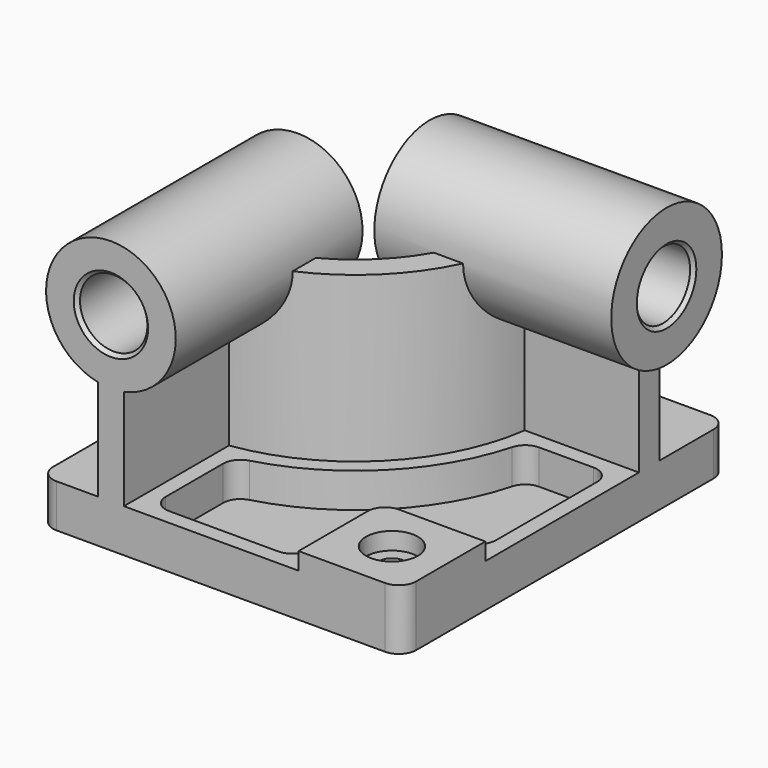
from build123d import *

# Parameters (mm, degrees)
F0_W            = 210
F0_H            = 225
F1_DEPTH        = 25
F3_DEPTH        = 95
F4_R            = 37.5
F5_DEPTH        = 10
F5_DEPTH_BACK   = 125
F6_R            = 40
F7_DEPTH        = 10
F7_DEPTH_BACK   = 127
F8_W            = 60
F8_H            = 60
F9_DEPTH        = 10
F10_R           = 10
F12_DEPTH       = 20
F14_D           = 15
F14_CBORE_D     = 30
F14_CBORE_DEPTH = 10
F15_R           = 10
F16_R           = 19.5
F17_DEPTH       = 235.001
F18_R           = 19.5
F19_DEPTH       = 220.001
F20_SIZE        = 2
F21_R           = 10


with BuildPart() as f1:
    # F0 (on Top) → F1 (new body)
    with BuildSketch(Plane.XY):
        Rectangle(F0_W, F0_H)
    extrude(amount=F1_DEPTH)

    # F2 (on face) → F3 (join)
    with BuildSketch(Plane.XY.offset(25)):
        with BuildLine():
            ThreePointArc((25, 63.5), (-3.1177490061, -4.3822509939), (-71, -32.5))
            Line((-71, -32.5), (-71, -112.5))
            Line((-71, -112.5), (-56, -112.5))
            Line((-56, -112.5), (-56, -46.4818166789))
            ThreePointArc((-56, -46.4818166789), (7.4888527117, -14.9888527117), (38.9818166789, 48.5))
            Line((38.9818166789, 48.5), (105, 48.5))
            Line((105, 48.5), (105, 63.5))
            Line((105, 63.5), (25, 63.5))
        make_face()
    extrude(amount=F3_DEPTH)

    # F4 (on face) → F5 (join, two sides)
    with BuildSketch(Plane.XZ.offset(112.5)) as f5_sk:
        with Locations((-63.5, 120)):
            Circle(F4_R)
        with BuildLine():
            ThreePointArc((-56, 83.2576538583), (-63.5, 82.5), (-71, 83.2576538583))
            Line((-71, 83.2576538583), (-71, 25))
            Line((-71, 25), (-105, 25))
            Line((-105, 25), (-105, 0))
            Line((-105, 0), (105, 0))
            Line((105, 0), (105, 25))
            Line((105, 25), (-56, 25))
            Line((-56, 25), (-56, 83.2576538583))
        make_face()
    extrude(amount=F5_DEPTH)
    extrude(f5_sk.sketch, amount=-F5_DEPTH_BACK)

    # F6 (on face) → F7 (join, two sides)
    with BuildSketch(Plane.YZ.offset(105)) as f7_sk:
        with Locations((56, 120)):
            Circle(F6_R)
        with BuildLine():
            ThreePointArc((63.5, 80.7094158862), (86.8220700148, 94.504902432), (96, 120))
            ThreePointArc((96, 120), (30.504902432, 150.8220700148), (48.5, 80.7094158862))
            Line((48.5, 80.7094158862), (48.5, 120))
            Line((48.5, 120), (63.5, 120))
            Line((63.5, 120), (63.5, 80.7094158862))
        make_face()
    extrude(amount=F7_DEPTH)
    extrude(f7_sk.sketch, amount=-F7_DEPTH_BACK)

    # F8 (on face) → F9 (join)
    with BuildSketch(Plane.XY.offset(25)):
        with Locations((75, -92.5)):
            Rectangle(F8_W, F8_H)
    extrude(amount=F9_DEPTH)

    # F10
    f10_edges = [f1.edges().sort_by_distance(p)[0] for p in [
        (45, -62.5, 30),
    ]]
    fillet(f10_edges, radius=F10_R)

    # F11 (on face) → F12 (cut)
    with BuildSketch(Plane.XY.offset(25)):
        with BuildLine():
            ThreePointArc((46.5755076536, 39.5), (13.8528137424, -21.3528137424), (-47, -54.0755076536))
            Line((-47, -54.0755076536), (-47, -113.5))
            Line((-47, -113.5), (36, -113.5))
            Line((36, -113.5), (36, -72.5))
            ThreePointArc((36, -72.5), (41.5649711575, -59.0649711575), (55, -53.5))
            Line((55, -53.5), (96, -53.5))
            Line((96, -53.5), (96, 39.5))
            Line((96, 39.5), (46.5755076536, 39.5))
        make_face()
    extrude(amount=-F12_DEPTH, mode=Mode.SUBTRACT)

    # F14 (through all)
    with Locations(Plane.XY.offset(35)):
        with Locations((75, -92.5)):
            CounterBoreHole(F14_D / 2, F14_CBORE_D / 2, F14_CBORE_DEPTH)

    # F15
    f15_edges = [f1.edges().sort_by_distance(p)[0] for p in [
        (-47, -54.075508, 15),
        (46.575508, 39.5, 15),
        (-47, -113.5, 15),
        (96, 39.5, 15),
        (96, -53.5, 15),
        (36, -113.5, 15),
    ]]
    fillet(f15_edges, radius=F15_R)

    # F16 (on face) → F17 (cut, through all)
    with BuildSketch(Plane.XZ.offset(122.5)):
        with Locations((-63.5, 120)):
            Circle(F16_R)
    extrude(amount=-F17_DEPTH, mode=Mode.SUBTRACT)

    # F18 (on face) → F19 (cut, through all)
    with BuildSketch(Plane.YZ.offset(115)):
        with Locations((56, 120)):
            Circle(F18_R)
    extrude(amount=-F19_DEPTH, mode=Mode.SUBTRACT)

    # F20
    f20_edges = [f1.edges().sort_by_distance(p)[0] for p in [
        (115, 36.5, 120),
        (-83, -122.5, 120),
        (-22, 36.5, 120),
        (-83, 12.5, 120),
    ]]
    chamfer(f20_edges, length=F20_SIZE)

    # F21
    f21_edges = [f1.edges().sort_by_distance(p)[0] for p in [
        (105, 112.5, 12.5),
        (105, -122.5, 17.5),
        (-105, 112.5, 12.5),
        (-105, -122.5, 12.5),
    ]]
    fillet(f21_edges, radius=F21_R)


solid = f1.part
